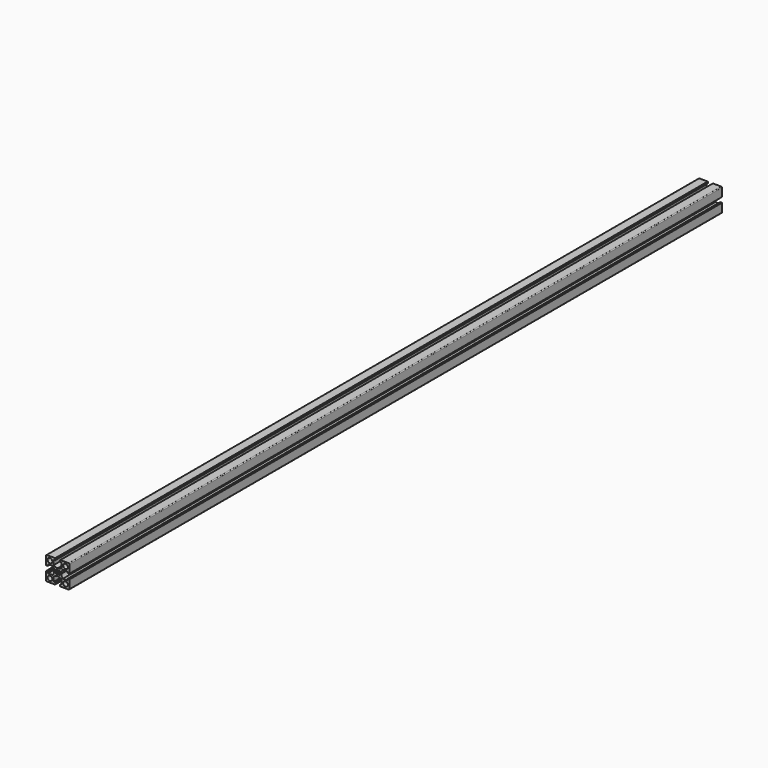
from build123d import *

# Parameters (mm, degrees)
F1_DEPTH = 1050


# Not quite as in the source:
# - ends of sketch curves that miss each other by under 0.0002 mm in the source are joined


with BuildPart() as f1:
    # F0 (on Front) → F1 (new body, symmetric)
    with BuildSketch(Plane.XZ):
        with BuildLine():
            Line((-15.716673, -9.862999), (-12.216673, -9.862999))
            ThreePointArc((-12.216673, -9.862999), (-12.0639163929, -8.6365278467), (-11.614980404, -7.4849973222))
            ThreePointArc((-11.614980404, -7.4849973222), (-11.5490626842, -7.1130153442), (-11.7185129313, -6.7753729313))
            Line((-11.7185129313, -6.7753729313), (-12.449264, -6.044623))
            ThreePointArc((-12.449264, -6.044623), (-12.625, -5.620359), (-12.4492640687, -5.1960949313))
            Line((-12.4492640687, -5.1960949313), (-12.166421, -4.913252))
            Line((-12.166421, -4.913252), (-11.883578, -4.630409))
            ThreePointArc((-11.883578, -4.630409), (-11.459314, -4.454673), (-11.0350499313, -4.6304089313))
            Line((-11.0350499313, -4.6304089313), (-10.3043, -5.361159))
            ThreePointArc((-10.3043, -5.361159), (-9.9666578911, -5.5306092814), (-9.5946760011, -5.4646919979))
            ThreePointArc((-9.5946760011, -5.4646919979), (-8.4431448102, -5.0157557733), (-7.216673, -4.862999))
            Line((-7.216673, -4.862999), (-7.216673, -1.362999))
            Line((-7.216673, -1.362999), (-7.725299, -0.854373))
            ThreePointArc((-7.725299, -0.854373), (-12.870898257, 0.243486803), (-17.3208396244, 3.0507114121))
            ThreePointArc((-17.3208396244, 3.0507114121), (-17.4655354529, 3.251778991), (-17.516673, 3.494163))
            Line((-17.516673, 3.494163), (-17.516673, 14.537001))
            ThreePointArc((-17.516673, 14.537001), (-17.3409370687, 14.9612650687), (-16.916673, 15.137001))
            Line((-16.916673, 15.137001), (-14.116673, 15.137001))
            ThreePointArc((-14.116673, 15.137001), (-13.6924089313, 15.3127369313), (-13.516673, 15.737001))
            Line((-13.516673, 15.737001), (-13.516673, 19.537001))
            ThreePointArc((-13.516673, 19.537001), (-13.6924089313, 19.9612650687), (-14.116673, 20.137001))
            Line((-14.116673, 20.137001), (-35.216673, 20.137001))
            ThreePointArc((-35.216673, 20.137001), (-36.6308865624, 19.5512145624), (-37.216673, 18.137001))
            Line((-37.216673, 18.137001), (-37.216673, -2.962999))
            ThreePointArc((-37.216673, -2.962999), (-37.0409370687, -3.3872630687), (-36.616673, -3.562999))
            Line((-36.616673, -3.562999), (-32.816673, -3.562999))
            ThreePointArc((-32.816673, -3.562999), (-32.3924089313, -3.3872630687), (-32.216673, -2.962999))
            Line((-32.216673, -2.962999), (-32.216673, -0.162999))
            ThreePointArc((-32.216673, -0.162999), (-32.0409370687, 0.2612650687), (-31.616673, 0.437001))
            Line((-31.616673, 0.437001), (-20.573835, 0.437001))
            ThreePointArc((-20.573835, 0.437001), (-20.3314509611, 0.3858634397), (-20.1303833502, 0.2411675922))
            ThreePointArc((-20.1303833502, 0.2411675922), (-17.3231587906, -4.2087737733), (-16.2252988273, -9.3543729941))
            Line((-16.2252988273, -9.3543729941), (-15.716673, -9.862999))
        make_face()
        with BuildLine():
            ThreePointArc((-27.216673, 16.137001), (-22.9740323129, 14.3796416871), (-21.216673, 10.137001))
            ThreePointArc((-21.216673, 10.137001), (-22.9740323129, 5.8943603129), (-27.216673, 4.137001))
            ThreePointArc((-27.216673, 4.137001), (-31.4593136871, 5.8943603129), (-33.216673, 10.137001))
            ThreePointArc((-33.216673, 10.137001), (-31.4593136871, 14.3796416871), (-27.216673, 16.137001))
        make_face(mode=Mode.SUBTRACT)
        with BuildLine():
            Line((-2.216673, -9.862999), (1.283327, -9.862999))
            Line((1.283327, -9.862999), (1.791952, -9.354373))
            ThreePointArc((1.791952, -9.354373), (2.8898126573, -4.208774101), (5.6970369143, 0.2411670781))
            ThreePointArc((5.6970369143, 0.2411670781), (5.898104653, 0.3858633036), (6.140489, 0.437001))
            Line((6.140489, 0.437001), (17.183327, 0.437001))
            ThreePointArc((17.183327, 0.437001), (17.6075910687, 0.2612650687), (17.783327, -0.162999))
            Line((17.783327, -0.162999), (17.783327, -2.962999))
            ThreePointArc((17.783327, -2.962999), (17.9590629313, -3.3872630687), (18.383327, -3.562999))
            Line((18.383327, -3.562999), (22.183327, -3.562999))
            ThreePointArc((22.183327, -3.562999), (22.6075910687, -3.3872630687), (22.783327, -2.962999))
            Line((22.783327, -2.962999), (22.783327, 10.137001))
            Line((22.783327, 10.137001), (22.783327, 18.137001))
            ThreePointArc((22.783327, 18.137001), (22.1975405624, 19.5512145624), (20.783327, 20.137001))
            Line((20.783327, 20.137001), (-0.316673, 20.137001))
            ThreePointArc((-0.316673, 20.137001), (-0.7409370687, 19.9612650687), (-0.916673, 19.537001))
            Line((-0.916673, 19.537001), (-0.916673, 15.737001))
            ThreePointArc((-0.916673, 15.737001), (-0.7409370687, 15.3127369313), (-0.316673, 15.137001))
            Line((-0.316673, 15.137001), (2.483327, 15.137001))
            ThreePointArc((2.483327, 15.137001), (2.9075910687, 14.9612650687), (3.083327, 14.537001))
            Line((3.083327, 14.537001), (3.083327, 3.494163))
            ThreePointArc((3.083327, 3.494163), (3.0321893036, 3.251778653), (2.8874930944, 3.0507108964))
            ThreePointArc((2.8874930944, 3.0507108964), (-1.5624485481, 0.2434864753), (-6.708047993, -0.8543732066))
            Line((-6.708047993, -0.8543732066), (-7.216673, -1.362999))
            Line((-7.216673, -1.362999), (-7.216673, -4.862999))
            ThreePointArc((-7.216673, -4.862999), (-5.9902016162, -5.0157556654), (-4.8386709038, -5.4646918222))
            ThreePointArc((-4.8386709038, -5.4646918222), (-4.4666891089, -5.5306092814), (-4.1290469313, -5.3611590687))
            Line((-4.1290469313, -5.3611590687), (-3.398297, -4.630409))
            ThreePointArc((-3.398297, -4.630409), (-2.974033, -4.454673), (-2.5497689313, -4.6304089313))
            Line((-2.5497689313, -4.6304089313), (-2.266926, -4.913252))
            Line((-2.266926, -4.913252), (-1.984083, -5.196095))
            ThreePointArc((-1.984083, -5.196095), (-1.808347, -5.620359), (-1.9840829313, -6.0446230687))
            Line((-1.9840829313, -6.0446230687), (-2.714833, -6.775373))
            ThreePointArc((-2.714833, -6.775373), (-2.8842832814, -7.1130151089), (-2.8183659979, -7.4849969989))
            ThreePointArc((-2.8183659979, -7.4849969989), (-2.7186094786, -7.6795557199), (-2.6274542351, -7.8782896692))
            ThreePointArc((-2.6274542351, -7.8782896692), (-2.3204451752, -8.8496120612), (-2.216673, -9.862999))
        make_face()
        with BuildLine():
            ThreePointArc((12.783327, 16.137001), (17.0259676871, 14.3796416871), (18.783327, 10.137001))
            ThreePointArc((18.783327, 10.137001), (17.0259676871, 5.8943603129), (12.783327, 4.137001))
            ThreePointArc((12.783327, 4.137001), (8.5406863129, 5.8943603129), (6.783327, 10.137001))
            ThreePointArc((6.783327, 10.137001), (8.5406863129, 14.3796416871), (12.783327, 16.137001))
        make_face(mode=Mode.SUBTRACT)
        with BuildLine():
            Line((1.791952, -10.371625), (1.283327, -9.862999))
            Line((1.283327, -9.862999), (-2.216673, -9.862999))
            ThreePointArc((-2.216673, -9.862999), (-2.3694296654, -11.0894703838), (-2.8183658222, -12.2410010962))
            ThreePointArc((-2.8183658222, -12.2410010962), (-2.8842833449, -12.6129834558), (-2.7148330687, -12.9506260687))
            Line((-2.7148330687, -12.9506260687), (-1.984083, -13.681376))
            ThreePointArc((-1.984083, -13.681376), (-1.808347, -14.10564), (-1.9840829313, -14.5299040687))
            Line((-1.9840829313, -14.5299040687), (-2.26692625, -14.81274675))
            Line((-2.26692625, -14.81274675), (-2.549769, -15.095589))
            ThreePointArc((-2.549769, -15.095589), (-2.974033, -15.271325), (-3.3982970687, -15.0955890687))
            Line((-3.3982970687, -15.0955890687), (-4.129047, -14.364839))
            ThreePointArc((-4.129047, -14.364839), (-4.4666891089, -14.1953887186), (-4.8386709989, -14.2613060021))
            ThreePointArc((-4.8386709989, -14.2613060021), (-5.9902016162, -14.7102423346), (-7.216673, -14.862999))
            Line((-7.216673, -14.862999), (-7.216673, -18.362999))
            Line((-7.216673, -18.362999), (-6.708048, -18.871625))
            ThreePointArc((-6.708048, -18.871625), (-1.5624482362, -19.9694846023), (2.887493576, -22.776709368))
            ThreePointArc((2.887493576, -22.776709368), (3.0321894397, -22.9777769611), (3.083327, -23.220161))
            Line((3.083327, -23.220161), (3.083327, -34.262999))
            ThreePointArc((3.083327, -34.262999), (2.9075910687, -34.6872630687), (2.483327, -34.862999))
            Line((2.483327, -34.862999), (-0.316673, -34.862999))
            ThreePointArc((-0.316673, -34.862999), (-0.7409370687, -35.0387349313), (-0.916673, -35.462999))
            Line((-0.916673, -35.462999), (-0.916673, -39.262999))
            ThreePointArc((-0.916673, -39.262999), (-0.7409370687, -39.6872630687), (-0.316673, -39.862999))
            Line((-0.316673, -39.862999), (20.783327, -39.862999))
            ThreePointArc((20.783327, -39.862999), (22.1975405624, -39.2772125624), (22.783327, -37.862999))
            Line((22.783327, -37.862999), (22.783327, -29.862999))
            Line((22.783327, -29.862999), (22.783327, -16.762999))
            ThreePointArc((22.783327, -16.762999), (22.6075910687, -16.3387349313), (22.183327, -16.162999))
            Line((22.183327, -16.162999), (18.383327, -16.162999))
            ThreePointArc((18.383327, -16.162999), (17.9590629313, -16.3387349313), (17.783327, -16.762999))
            Line((17.783327, -16.762999), (17.783327, -19.562999))
            ThreePointArc((17.783327, -19.562999), (17.6075910687, -19.9872630687), (17.183327, -20.162999))
            Line((17.183327, -20.162999), (6.140489, -20.162999))
            ThreePointArc((6.140489, -20.162999), (5.898104991, -20.1118614529), (5.6970373943, -19.9671656406))
            ThreePointArc((5.6970373943, -19.9671656406), (2.8898127966, -15.5172242413), (1.791952, -10.371625))
        make_face()
        with BuildLine():
            ThreePointArc((12.783327, -23.862999), (17.0259676871, -25.6203583129), (18.783327, -29.862999))
            ThreePointArc((18.783327, -29.862999), (17.0259676871, -34.1056396871), (12.783327, -35.862999))
            ThreePointArc((12.783327, -35.862999), (8.5406863129, -34.1056396871), (6.783327, -29.862999))
            ThreePointArc((6.783327, -29.862999), (8.5406863129, -25.6203583129), (12.783327, -23.862999))
        make_face(mode=Mode.SUBTRACT)
        with BuildLine():
            Line((-7.216673, -18.362999), (-7.216673, -14.862999))
            ThreePointArc((-7.216673, -14.862999), (-8.4431448102, -14.7102422267), (-9.59467587, -14.2613057595))
            ThreePointArc((-9.59467587, -14.2613057595), (-9.9666578911, -14.1953887186), (-10.3043000687, -14.3648389313))
            Line((-10.3043000687, -14.3648389313), (-11.03505, -15.095589))
            ThreePointArc((-11.03505, -15.095589), (-11.459314, -15.271325), (-11.8835780687, -15.0955890687))
            Line((-11.8835780687, -15.0955890687), (-12.16642075, -14.81274675))
            Line((-12.16642075, -14.81274675), (-12.449264, -14.529904))
            ThreePointArc((-12.449264, -14.529904), (-12.625, -14.10564), (-12.4492640687, -13.6813759313))
            Line((-12.4492640687, -13.6813759313), (-11.718513, -12.950626))
            ThreePointArc((-11.718513, -12.950626), (-11.5490626207, -12.6129832205), (-11.6149806466, -12.2410008089))
            ThreePointArc((-11.6149806466, -12.2410008089), (-11.7147367119, -12.0464418876), (-11.8058919225, -11.8477079665))
            Line((-11.8058919225, -11.8477079665), (-13.366227, -12.522509))
            Line((-13.366227, -12.522509), (-16.8006937252, -14.0078200514))
            ThreePointArc((-16.8006937252, -14.0078200514), (-18.1220223785, -17.1794274389), (-20.1303838659, -19.9671661223))
            ThreePointArc((-20.1303838659, -19.9671661223), (-20.3314512991, -20.1118615889), (-20.573835, -20.162999))
            Line((-20.573835, -20.162999), (-31.0332393373, -20.162999))
            Line((-31.0332393373, -20.162999), (-37.216673, -22.8371615671))
            Line((-37.216673, -22.8371615671), (-37.216673, -37.862999))
            ThreePointArc((-37.216673, -37.862999), (-36.6308865624, -39.2772125624), (-35.216673, -39.862999))
            Line((-35.216673, -39.862999), (-14.116673, -39.862999))
            ThreePointArc((-14.116673, -39.862999), (-13.6924089313, -39.6872630687), (-13.516673, -39.262999))
            Line((-13.516673, -39.262999), (-13.516673, -35.462999))
            ThreePointArc((-13.516673, -35.462999), (-13.6924089313, -35.0387349313), (-14.116673, -34.862999))
            Line((-14.116673, -34.862999), (-16.916673, -34.862999))
            ThreePointArc((-16.916673, -34.862999), (-17.3409370687, -34.6872630687), (-17.516673, -34.262999))
            Line((-17.516673, -34.262999), (-17.516673, -23.220161))
            ThreePointArc((-17.516673, -23.220161), (-17.4655355889, -22.9777772991), (-17.3208401385, -22.7767098481))
            ThreePointArc((-17.3208401385, -22.7767098481), (-12.870898569, -19.9694849299), (-7.7252990059, -18.8716248273))
            Line((-7.7252990059, -18.8716248273), (-7.216673, -18.362999))
        make_face()
        with BuildLine():
            ThreePointArc((-27.216673, -23.862999), (-22.9740323129, -25.6203583129), (-21.216673, -29.862999))
            ThreePointArc((-21.216673, -29.862999), (-22.9740323129, -34.1056396871), (-27.216673, -35.862999))
            ThreePointArc((-27.216673, -35.862999), (-31.4593136871, -34.1056396871), (-33.216673, -29.862999))
            ThreePointArc((-33.216673, -29.862999), (-31.4593136871, -25.6203583129), (-27.216673, -23.862999))
        make_face(mode=Mode.SUBTRACT)
        with BuildLine():
            ThreePointArc((-11.8058919225, -11.8477079665), (-12.112900865, -10.8763857444), (-12.216673, -9.862999))
            Line((-12.216673, -9.862999), (-15.716673, -9.862999))
            Line((-15.716673, -9.862999), (-16.225299, -10.371625))
            ThreePointArc((-16.225299, -10.371625), (-16.4010195281, -12.2074418337), (-16.8006937252, -14.0078200514))
            Line((-16.8006937252, -14.0078200514), (-13.366227, -12.522509))
            Line((-13.366227, -12.522509), (-11.8058919225, -11.8477079665))
        make_face()
        with BuildLine():
            Line((-37.216673, -22.8371615671), (-31.0332393373, -20.162999))
            Line((-31.0332393373, -20.162999), (-31.616673, -20.162999))
            ThreePointArc((-31.616673, -20.162999), (-32.0409370687, -19.9872630687), (-32.216673, -19.562999))
            Line((-32.216673, -19.562999), (-32.216673, -16.762999))
            ThreePointArc((-32.216673, -16.762999), (-32.3924089313, -16.3387349313), (-32.816673, -16.162999))
            Line((-32.816673, -16.162999), (-36.616673, -16.162999))
            ThreePointArc((-36.616673, -16.162999), (-37.0409370687, -16.3387349313), (-37.216673, -16.762999))
            Line((-37.216673, -16.762999), (-37.216673, -22.8371615671))
        make_face()
    extrude(amount=F1_DEPTH, both=True)


solid = f1.part
